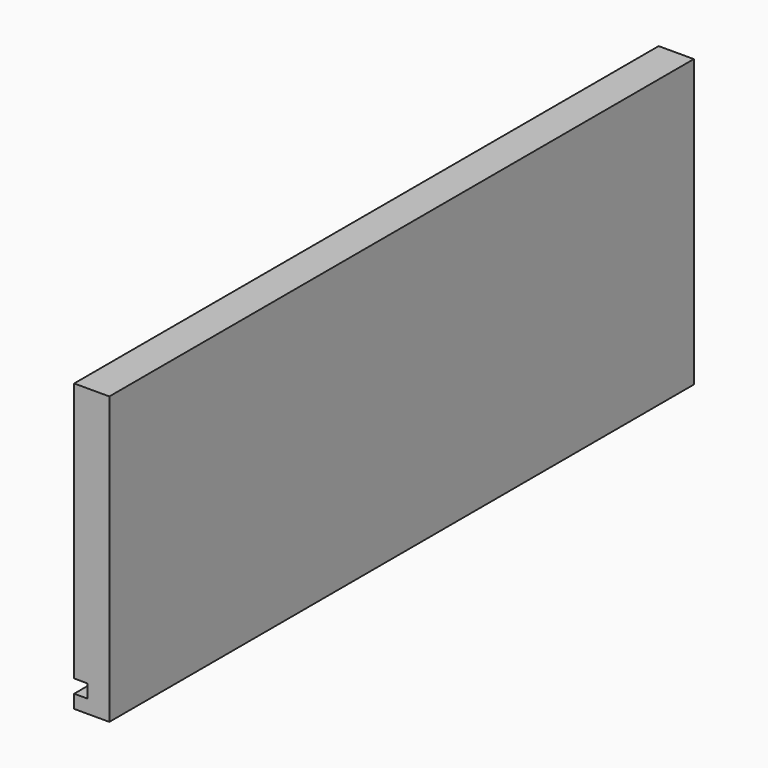
from build123d import *

# Parameters (mm, degrees)
F4_DEPTH = 346.1004


# Not quite as in the source:
# - a variable given as a bare number and used for a length is read in inches; the dataset says mm whatever the document's units were


with BuildPart() as f4:
    # F3 (on Front) → F4 (new body)
    with BuildSketch(Plane.XZ):
        Polygon((-16.6624, 0), (0, 0), (0, 135.7376), (-16.6624, 135.7376), (-16.6624, 12.7), (-10.3124, 12.7), (-10.3124, 6.35), (-16.6624, 6.35), align=None)
    extrude(amount=F4_DEPTH)


solid = f4.part
